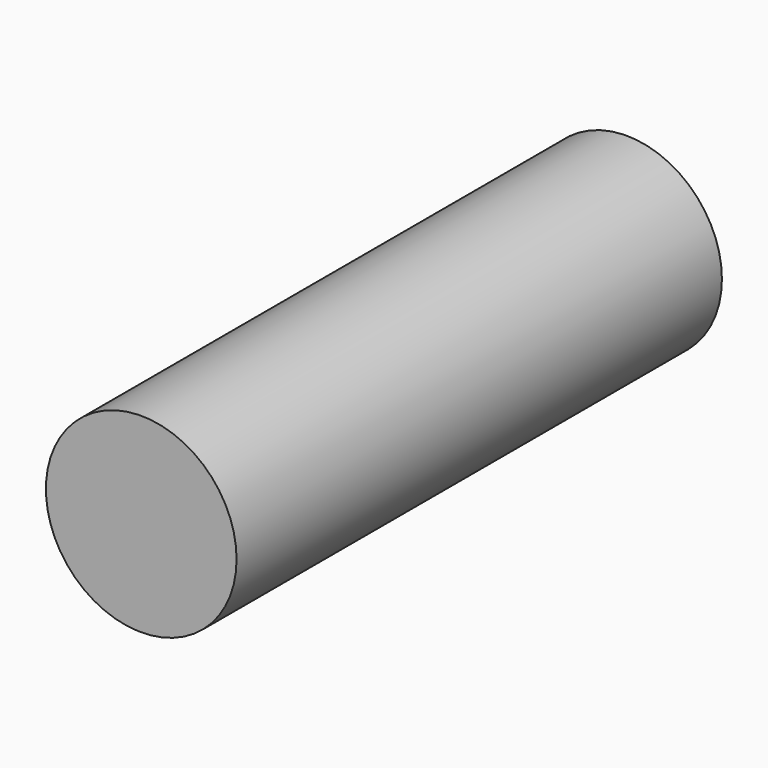
from build123d import *

# Parameters (mm, degrees)
F0_R     = 13.97
F2_DEPTH = 88.9
F1_R     = 1.5875
F3_DEPTH = 142


# Not quite as in the source:
# - an extrude ends at something that could not be found from the text; its depth is read off the source's solid


with BuildPart() as f2:
    # F0 (on Front) → F2 (new body)
    with BuildSketch(Plane.XZ):
        Circle(F0_R)
    extrude(amount=F2_DEPTH)

    # F1 (on Front) → F3 (cut, through all)
    with BuildSketch(Plane.XZ):
        Circle(F1_R)
    extrude(amount=-F3_DEPTH, mode=Mode.SUBTRACT)


solid = f2.part
